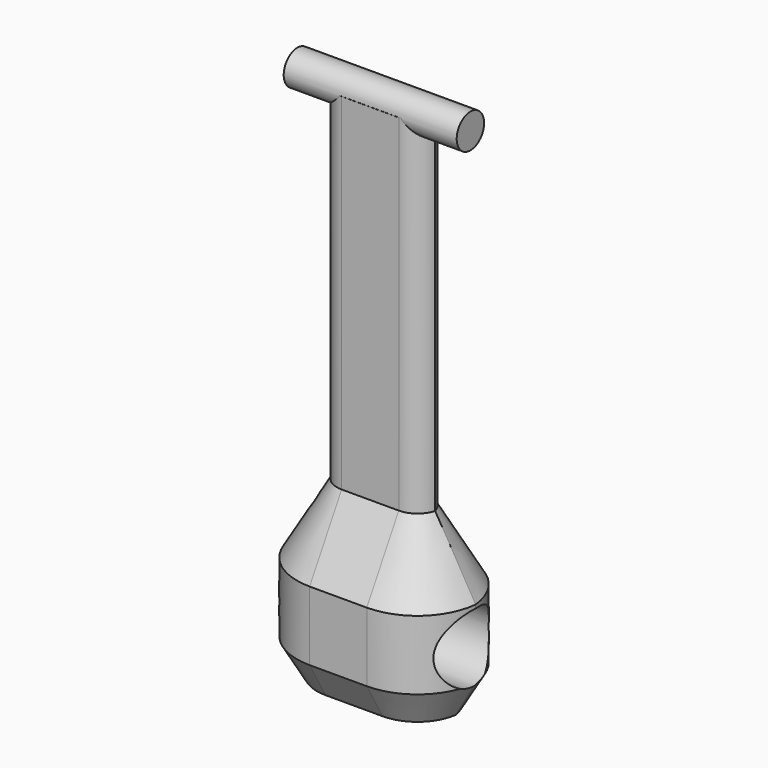
from build123d import *

# Parameters (mm, degrees)
F0_R                   = 0.2475329231
F1_DEPTH               = 2.5
F2_W                   = 1.5014072414
F2_H                   = 0.4986668355
F3_DEPTH               = 5
F4_T4_DEPTH            = 6.6899494937
F4_S5_R                = 0.2475329231
F4_T6_DEPTH            = 5
F4_T10_DEPTH           = 6.6899494937
F4_S11_R               = 0.2475329231
F4_T12_DEPTH           = 5
F4_T16_DEPTH           = 6.6899494937
F4_S17_R               = 0.2475329231
F4_T18_DEPTH           = 5
F4_T22_DEPTH           = 6.6899494937
F4_S23_R               = 0.2475329231
F4_T24_DEPTH           = 5
F5_DEPTH               = 1
DRAFT_F5_DRAFTED_ANGLE = -30
F6_DEPTH               = 1
F7_DEPTH               = 0.5
DRAFT_F7_DRAFTED_ANGLE = 30
F9_D                   = 1
F9_DEPTH               = 2.5761580853
F11_D                  = 1
F11_DEPTH              = 0.0733426202


# Not quite as in the source:
# - a fillet or chamfer that OpenCascade refuses, or shapes differently, is made with other operations: its cross-section is extruded or revolved along the edge and cut away or added
# - an extrude with a draft is written as a straight extrude whose walls are then drafted


with BuildPart() as f1:
    # F0 (on Right) → F1 (new body)
    with BuildSketch(Plane.YZ):
        Circle(F0_R)
    extrude(amount=F1_DEPTH)

    # F2 (on Top) → F3 (join)
    with BuildSketch(Plane.XY):
        with Locations((1.2514077825, 0)):
            Rectangle(F2_W, F2_H)
    extrude(amount=-F3_DEPTH)

    # F4: fillet of radius 0.3379898987 on 4 edges, made by hand


with BuildPart() as f4_tool2:
    # F4_s3 → F4_t4 (new body)
    with BuildSketch(Plane.XY.offset(0.8449747468)):
        with BuildLine():
            ThreePointArc((0.5007041618, 0.088656481), (0.5996991112, -0.1503384684), (0.8386940606, -0.2493334177))
            Line((0.8386940606, -0.2493334177), (0.5007041618, -0.2493334177))
            Line((0.5007041618, -0.2493334177), (0.5007041618, 0.088656481))
        make_face()
    extrude(amount=-F4_T4_DEPTH)

    # F4_s5 → F4_t6 (cut, symmetric)
    with BuildSketch(Plane.YZ.offset(0.7)):
        Circle(F4_S5_R)
    extrude(amount=F4_T6_DEPTH, both=True, mode=Mode.SUBTRACT)


with BuildPart() as f1_1:
    add(f1.part)

    # F4_t1: cut F4_tool2
    add(f4_tool2.part, mode=Mode.SUBTRACT)


with BuildPart() as f4_tool8:
    # F4_s9 → F4_t10 (new body)
    with BuildSketch(Plane.XY.offset(0.8449747468)):
        with BuildLine():
            ThreePointArc((0.5007041618, -0.088656481), (0.5996991112, 0.1503384684), (0.8386940606, 0.2493334177))
            Line((0.8386940606, 0.2493334177), (0.5007041618, 0.2493334177))
            Line((0.5007041618, 0.2493334177), (0.5007041618, -0.088656481))
        make_face()
    extrude(amount=-F4_T10_DEPTH)

    # F4_s11 → F4_t12 (cut, symmetric)
    with BuildSketch(Plane.YZ.offset(0.7)):
        Circle(F4_S11_R)
    extrude(amount=F4_T12_DEPTH, both=True, mode=Mode.SUBTRACT)


with BuildPart() as f1_2:
    add(f1_1.part)

    # F4_t7: cut F4_tool8
    add(f4_tool8.part, mode=Mode.SUBTRACT)


with BuildPart() as f4_tool14:
    # F4_s15 → F4_t16 (new body)
    with BuildSketch(Plane.XY.offset(0.8449747468)):
        with BuildLine():
            ThreePointArc((2.0021114033, -0.088656481), (1.9031164539, 0.1503384684), (1.6641215045, 0.2493334177))
            Line((1.6641215045, 0.2493334177), (2.0021114033, 0.2493334177))
            Line((2.0021114033, 0.2493334177), (2.0021114033, -0.088656481))
        make_face()
    extrude(amount=-F4_T16_DEPTH)

    # F4_s17 → F4_t18 (cut, symmetric)
    with BuildSketch(Plane.YZ.offset(1.8)):
        Circle(F4_S17_R)
    extrude(amount=F4_T18_DEPTH, both=True, mode=Mode.SUBTRACT)


with BuildPart() as f1_3:
    add(f1_2.part)

    # F4_t13: cut F4_tool14
    add(f4_tool14.part, mode=Mode.SUBTRACT)


with BuildPart() as f4_tool20:
    # F4_s21 → F4_t22 (new body)
    with BuildSketch(Plane.XY.offset(0.8449747468)):
        with BuildLine():
            ThreePointArc((2.0021114033, 0.088656481), (1.9031164539, -0.1503384684), (1.6641215045, -0.2493334177))
            Line((1.6641215045, -0.2493334177), (2.0021114033, -0.2493334177))
            Line((2.0021114033, -0.2493334177), (2.0021114033, 0.088656481))
        make_face()
    extrude(amount=-F4_T22_DEPTH)

    # F4_s23 → F4_t24 (cut, symmetric)
    with BuildSketch(Plane.YZ.offset(1.8)):
        Circle(F4_S23_R)
    extrude(amount=F4_T24_DEPTH, both=True, mode=Mode.SUBTRACT)


with BuildPart() as f1_4:
    add(f1_3.part)

    # F4_t19: cut F4_tool20
    add(f4_tool20.part, mode=Mode.SUBTRACT)


with BuildPart() as f5_drafted:
    # F5 (new): a face of the model
    f5_faces = [f1_4.part.faces().sort_by_distance(p)[0] for p in [
        (1.2514077826, 0, -5),
    ]]
    extrude(f5_faces, amount=F5_DEPTH)

    # draft_F5_drafted
    draft_f5_drafted_walls = [f5_drafted.faces().sort_by_distance(p)[0] for p in [
        (1.2514077825, 0.2493334177, -5.6666666667),
        (1.8693922728, 0.1798599679, -5.6666666667),
        (1.8693922728, -0.1798599679, -5.6666666667),
        (1.2514077825, -0.2493334177, -5.6666666667),
        (0.6334232923, -0.1798599679, -5.6666666667),
        (0.6334232923, 0.1798599679, -5.6666666667),
    ]]
    draft(draft_f5_drafted_walls, neutral_plane=Plane(origin=(1.2514077826, 0, -5), x_dir=(1, 0, 0), z_dir=(0, 0, -1)), angle=DRAFT_F5_DRAFTED_ANGLE)


with BuildPart() as f1_5:
    add(f1_4.part)

    # join_F5_drafted: union F5_drafted
    add(f5_drafted.part)

    # F6 (add): a face of the model
    f6_faces = [f1_5.faces().sort_by_distance(p)[0] for p in [
        (1.2514077825, 0, -6),
    ]]
    extrude(f6_faces, amount=F6_DEPTH)


with BuildPart() as f7_drafted:
    # F7 (new): a face of the model
    f7_faces = [f1_5.part.faces().sort_by_distance(p)[0] for p in [
        (1.2514077825, 0, -7),
    ]]
    extrude(f7_faces, amount=F7_DEPTH)

    # draft_F7_drafted
    draft_f7_drafted_walls = [f7_drafted.faces().sort_by_distance(p)[0] for p in [
        (1.2514077825, 0.8266836869, -7.3333333333),
        (2.2792218154, 0.5892072447, -7.3333333333),
        (2.2792218153, -0.5892072448, -7.3333333333),
        (1.2514077824, -0.8266836869, -7.3333333333),
        (0.2235937497, -0.5892072447, -7.3333333333),
        (0.2235937497, 0.5892072447, -7.3333333333),
    ]]
    draft(draft_f7_drafted_walls, neutral_plane=Plane(origin=(1.2514077825, 0, -7), x_dir=(1, 0, 0), z_dir=(0, 0, -1)), angle=DRAFT_F7_DRAFTED_ANGLE)


with BuildPart() as f1_6:
    add(f1_5.part)

    # join_F7_drafted: union F7_drafted
    add(f7_drafted.part)

    # F9 (through all, one way)
    with BuildSketch(Plane(origin=(0, 0, 0), x_dir=(0, 1, 0), z_dir=(-1, 0, 0))):
        with Locations((0, 6.5516633913)):
            Circle(F9_D / 2)
    extrude(amount=-F9_DEPTH, mode=Mode.SUBTRACT)

    # F11 (through all, one way)
    with BuildSketch(Plane.YZ):
        with Locations((0, -6.5546627156)):
            Circle(F11_D / 2)
    extrude(amount=-F11_DEPTH, mode=Mode.SUBTRACT)


solid = f1_6.part
